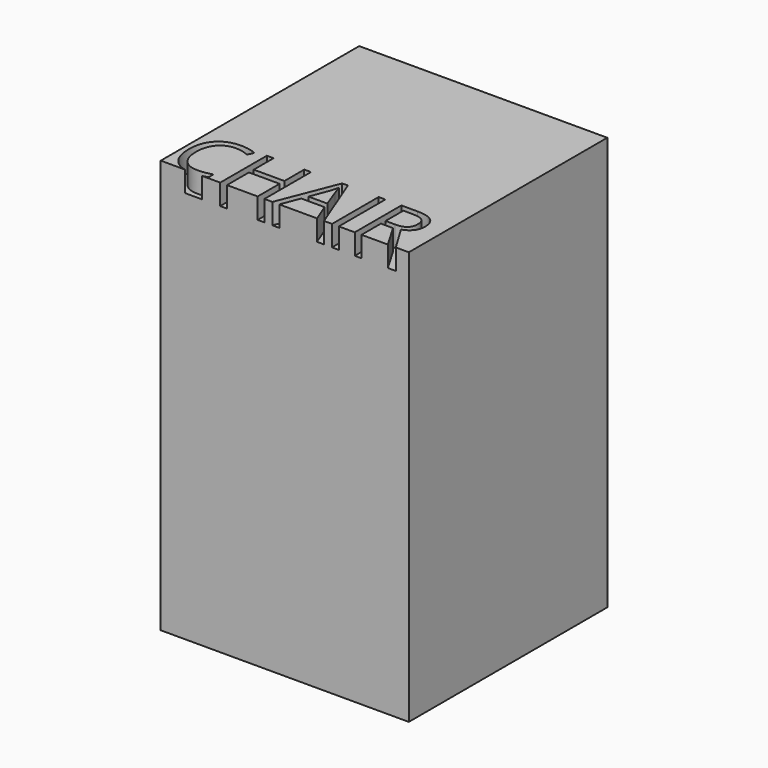
from build123d import *

# Parameters (mm, degrees)
F0_W         = 300
F0_H         = 300
F1_DEPTH     = 500
F2_TEXT_SIZE = 98.6526483239
F3_DEPTH     = 25


# Not quite as in the source:
# - Text() gives the source's letters only with a copy of the font that has no kerning and outlines rounded to 1/6400 em; it was checked with that copy


with BuildPart() as f1:
    # F0 (on Top) → F1 (new body)
    with BuildSketch(Plane.XY):
        Rectangle(F0_W, F0_H)
    extrude(amount=F1_DEPTH)

    # F2 (on face) → F3 (cut)
    with BuildSketch(Plane.XY.offset(500)):
        with Locations((-150, -150)):
            Text('CHAIR', F2_TEXT_SIZE, font='Open Sans', text_align=(TextAlign.LEFT, TextAlign.BOTTOM))
    extrude(amount=-F3_DEPTH, mode=Mode.SUBTRACT)


solid = f1.part
